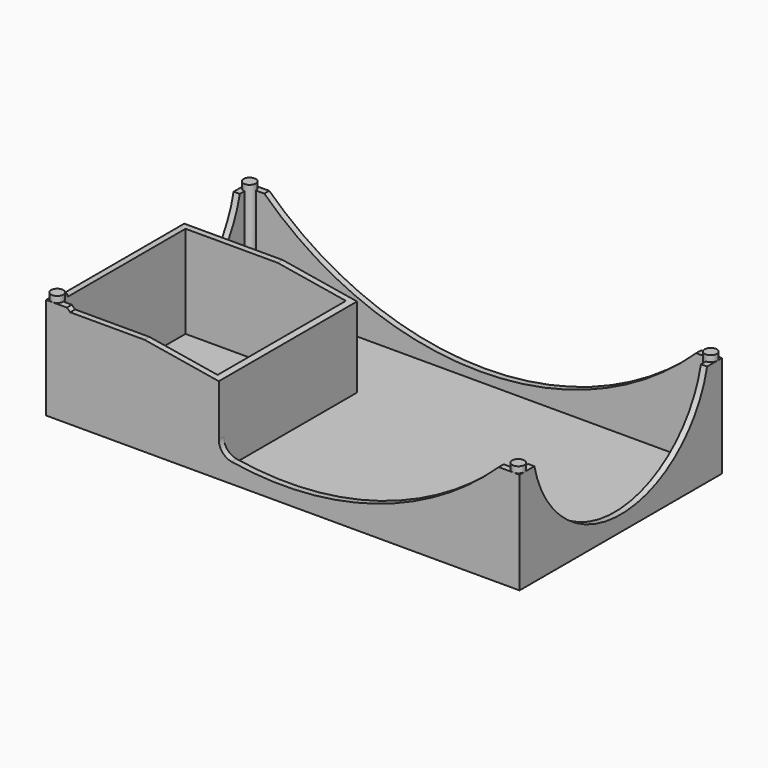
from build123d import *

# Parameters (mm, degrees)
F0_W      = 153.5
F0_H      = 82
F1_DEPTH  = 2
F2_R      = 7
F2_R_2    = 1.75
F3_DEPTH  = 2.001
F4_SIZE   = 1.99999
F5_R      = 2
F6_DEPTH  = 33
F7_W      = 153.5
F7_H      = 82
F7_W_2    = 149.5
F7_H_2    = 78
F8_DEPTH  = 31
F10_DEPTH = 82.001
F12_DEPTH = 153.501
F13_W     = 56
F13_H     = 56
F13_W_2   = 52
F13_H_2   = 52
F14_DEPTH = 30
F16_DEPTH = 82.001
F17_R     = 5


# Not quite as in the source:
# - a fillet or chamfer is up to 0.001 mm smaller than in the source, because OpenCascade refuses the exact size


with BuildPart() as f1:
    # F0 (on Top) → F1 (new body)
    with BuildSketch(Plane.XY):
        Rectangle(F0_W, F0_H)
    extrude(amount=F1_DEPTH)

    # F2 (on face) → F3 (cut, through all)
    with BuildSketch(Plane.XY.offset(2)):
        with Locations((-48.75, -13)):
            Circle(F2_R)
        with Locations((-68.75, -13)):
            Circle(F2_R_2)
        with Locations((-28.75, -13)):
            Circle(F2_R_2)
    extrude(amount=-F3_DEPTH, mode=Mode.SUBTRACT)

    # F4 (size 2 in the source; OpenCascade refuses exactly that, so slightly less here)
    f4_edges = [f1.edges().sort_by_distance(p)[0] for p in [
        (-70.5, -13, 0),
        (-30.5, -13, 0),
    ]]
    chamfer(f4_edges, length=F4_SIZE)

    # F5 (on face) → F6 (join)
    with BuildSketch(Plane.XY.offset(2)):
        with Locations((-74.75, 39)):
            Circle(F5_R)
        with Locations((74.75, 39)):
            Circle(F5_R)
        with Locations((-74.75, -39)):
            Circle(F5_R)
        with Locations((74.75, -39)):
            Circle(F5_R)
    extrude(amount=F6_DEPTH)

    # F7 (on face) → F8 (join)
    with BuildSketch(Plane.XY.offset(2)):
        Rectangle(F7_W, F7_H)
        Rectangle(F7_W_2, F7_H_2, mode=Mode.SUBTRACT)
    extrude(amount=F8_DEPTH)

    # F9 (on face) → F10 (cut, through all)
    with BuildSketch(Plane.XZ.offset(41)):
        with BuildLine():
            Line((70, 33), (-70, 33))
            ThreePointArc((-70, 33), (0, 5), (70, 33))
        make_face()
    extrude(amount=-F10_DEPTH, mode=Mode.SUBTRACT)

    # F11 (on face) → F12 (cut, through all)
    with BuildSketch(Plane.YZ.offset(76.75)):
        with BuildLine():
            Line((35, 33), (-35, 33))
            ThreePointArc((-35, 33), (0, 5), (35, 33))
        make_face()
    extrude(amount=-F12_DEPTH, mode=Mode.SUBTRACT)

    # F13 (on face) → F14 (join)
    with BuildSketch(Plane.XY.offset(2)):
        with Locations((-48.75, -13)):
            Rectangle(F13_W, F13_H)
        with Locations((-48.75, -13)):
            Rectangle(F13_W_2, F13_H_2, mode=Mode.SUBTRACT)
    extrude(amount=F14_DEPTH)

    # F15 (on face) → F16 (cut, through all)
    with BuildSketch(Plane.XZ.offset(41)):
        Polygon((-20.75, 28), (-20.75, 32), (-44.8423758792, 32), align=None)
    extrude(amount=-F16_DEPTH, mode=Mode.SUBTRACT)

    # F17
    f17_edges = [f1.edges().sort_by_distance(p)[0] for p in [
        (-20.75, -40, 7.143634),
        (-75.75, 15, 8.286419),
    ]]
    fillet(f17_edges, radius=F17_R)


solid = f1.part
